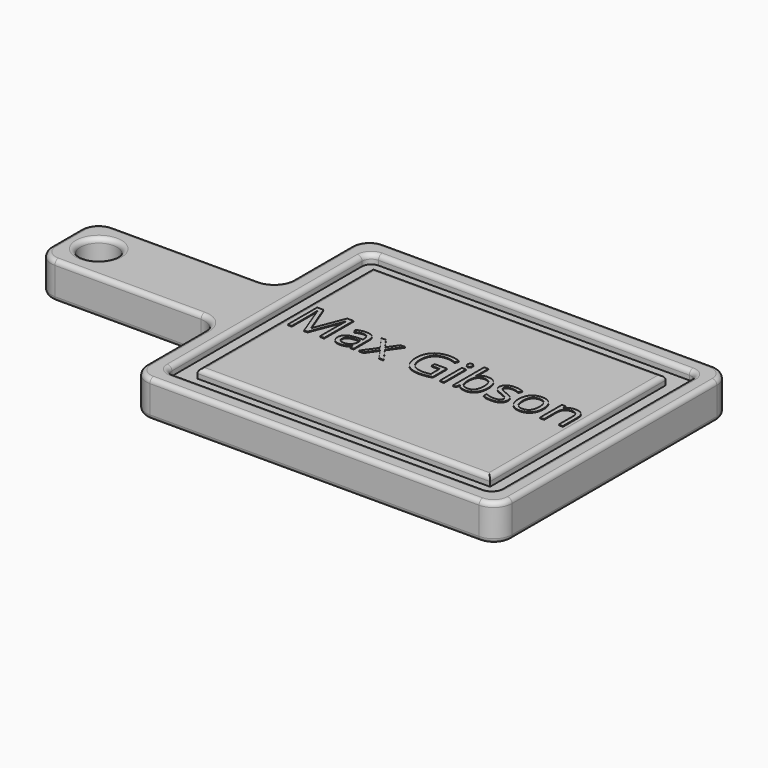
from build123d import *

# Parameters (mm, degrees)
F0_W         = 127
F0_H         = 50.8
F1_DEPTH     = 25.4
F2_R         = 12.7
F3_DEPTH     = 25.4
F5_DEPTH     = 6.35
F6_R         = 6.35
F7_R         = 12.7
F8_R         = 3.175
F9_TEXT_SIZE = 35.6895183099
F10_DEPTH    = 0.508


# Not quite as in the source:
# - Text() gives the source's letters only with a copy of the font that has no kerning and outlines rounded to 1/6400 em; it was checked with that copy


with BuildPart() as f1:
    # F0 (on Top) → F1 (new body)
    with BuildSketch(Plane.XY):
        Polygon((0, 76.2), (0, 0), (254, 0), (254, 203.2), (0, 203.2), (0, 127), align=None)
        with Locations((-63.5, 101.6)):
            Rectangle(F0_W, F0_H)
    extrude(amount=F1_DEPTH)

    # F2 (on face) → F3 (cut)
    with BuildSketch(Plane.XY.offset(25.4)):
        with Locations((-104.14, 101.6)):
            Circle(F2_R)
    extrude(amount=-F3_DEPTH, mode=Mode.SUBTRACT)

    # F4 (on face) → F5 (cut)
    with BuildSketch(Plane.XY.offset(25.4)):
        Polygon((12.6999939203, 76.2), (12.6999939203, 12.6999939203), (241.3000060797, 12.6999939203), (241.3000060797, 190.5000060797), (12.6999939203, 190.5000060797), (12.6999939203, 127), align=None)
        Polygon((25.4000002861, 76.2), (25.4000002861, 127), (25.4000002861, 177.7999997139), (228.5999997139, 177.7999997139), (228.5999997139, 25.4000002861), (25.4000002861, 25.4000002861), align=None, mode=Mode.SUBTRACT)
    extrude(amount=-F5_DEPTH, mode=Mode.SUBTRACT)

    # F6
    f6_edges = [f1.edges().sort_by_distance(p)[0] for p in [
        (12.699994, 190.500006, 22.225),
        (241.300006, 190.500006, 22.225),
        (241.300006, 12.699994, 22.225),
        (12.699994, 12.699994, 22.225),
    ]]
    fillet(f6_edges, radius=F6_R)

    # F7
    f7_edges = [f1.edges().sort_by_distance(p)[0] for p in [
        (0, 203.2, 12.7),
        (-127, 127, 12.7),
        (-127, 76.2, 12.7),
        (0, 0, 12.7),
        (254, 0, 12.7),
        (254, 203.2, 12.7),
        (0, 76.2, 12.7),
        (0, 127, 12.7),
    ]]
    fillet(f7_edges, radius=F7_R)

    # F8
    f8_edges = [f1.edges().sort_by_distance(p)[0] for p in [
        (127, 177.8, 25.4),
        (228.6, 101.6, 25.4),
        (127, 25.4, 25.4),
        (25.4, 101.6, 25.4),
        (0, 38.1, 25.4),
        (-3.719744, 72.480256, 25.4),
        (3.719744, 3.719744, 25.4),
        (-63.5, 76.2, 25.4),
        (127, 0, 25.4),
        (-123.280256, 79.919744, 25.4),
        (250.280256, 3.719744, 25.4),
        (-127, 101.6, 25.4),
        (254, 101.6, 25.4),
        (-123.280256, 123.280256, 25.4),
        (250.280256, 199.480256, 25.4),
        (-63.5, 127, 25.4),
        (127, 203.2, 25.4),
        (-3.719744, 130.719744, 25.4),
        (3.719744, 199.480256, 25.4),
        (0, 165.1, 25.4),
        (127, 12.699994, 25.4),
        (14.559866, 14.559866, 25.4),
        (239.440134, 14.559866, 25.4),
        (12.699994, 101.6, 25.4),
        (241.300006, 101.6, 25.4),
        (14.559866, 188.640134, 25.4),
        (239.440134, 188.640134, 25.4),
        (127, 190.500006, 25.4),
        (-116.84, 101.6, 25.4),
        (0, 38.1, 0),
        (-3.719744, 72.480256, 0),
        (3.719744, 3.719744, 0),
        (-63.5, 76.2, 0),
        (127, 0, 0),
        (-123.280256, 79.919744, 0),
        (250.280256, 3.719744, 0),
        (-127, 101.6, 0),
        (254, 101.6, 0),
        (-123.280256, 123.280256, 0),
        (250.280256, 199.480256, 0),
        (-63.5, 127, 0),
        (127, 203.2, 0),
        (-3.719744, 130.719744, 0),
        (3.719744, 199.480256, 0),
        (0, 165.1, 0),
        (-116.84, 101.6, 0),
    ]]
    fillet(f8_edges, radius=F8_R)

    # F9 (on face) → F10 (join)
    with BuildSketch(Plane.XY.offset(25.4)):
        with Locations((28.5750002861, 95.5232417487)):
            Text('Max Gibson', F9_TEXT_SIZE, font='Open Sans', text_align=(TextAlign.LEFT, TextAlign.BOTTOM))
    extrude(amount=F10_DEPTH)


solid = f1.part
